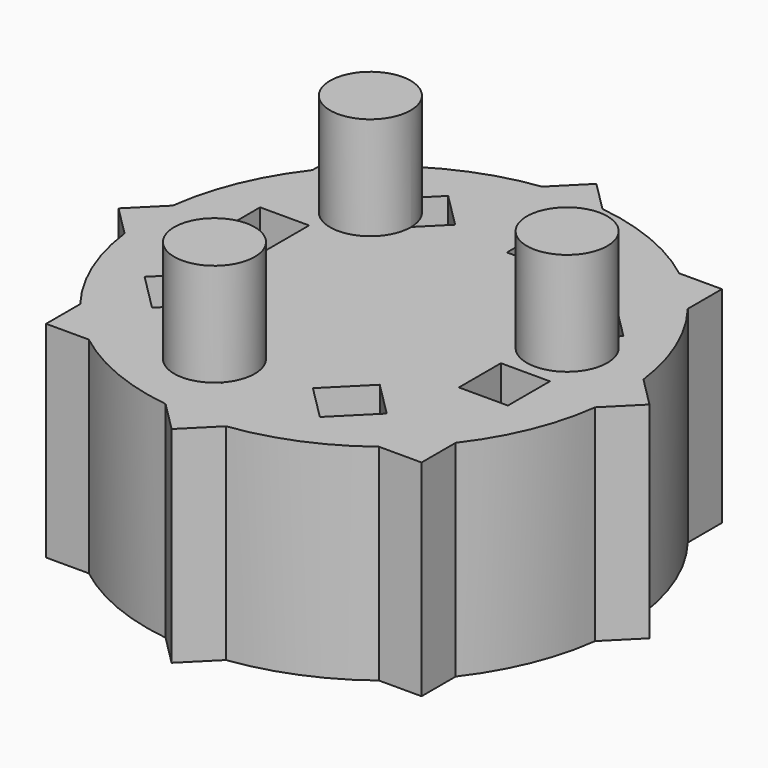
from build123d import *

# Parameters (mm, degrees)
F0_R            = 58.5548573359
F1_DEPTH        = 25.4
F2_R            = 9.9387856365
F3_DEPTH        = 25.4
F3_COPIES_COUNT = 3
F5_DEPTH        = 50.8
F5_COPIES_COUNT = 8
F6_W            = 12.9660330713
F6_H            = 12.1016278863
F7_DEPTH        = 25.4
F7_COPIES_COUNT = 8


# Not quite as in the source:
# - a pattern or mirror of a feature is missing from the dataset's text; its kind, count and spacing are read off the source's solid


with BuildPart() as f1:
    # F0 (on Top) → F1 (new body, symmetric)
    with BuildSketch(Plane.XY):
        Circle(F0_R)
    extrude(amount=F1_DEPTH, both=True)

    # F2 (on face) → F3 (join)
    with BuildSketch(Plane.XY.offset(25.4)):
        with Locations((-26.5582595021, 29.0003977716)):
            Circle(F2_R)
    f3 = extrude(amount=F3_DEPTH)

    # F3_copies: F3 ×3 about axis
    f3_copies_axis = Axis((0, 0, 0), (0, 0, 1))
    for i in range(1, F3_COPIES_COUNT):
        add(f3.rotate(f3_copies_axis, i * 360 / F3_COPIES_COUNT))

    # F4 (on face) → F5 (join, through all)
    with BuildSketch(Plane.XY.offset(25.4)):
        with BuildLine():
            Line((0, 65.528380896), (-7.4493038573, 58.0790770387))
            ThreePointArc((-7.4493038573, 58.0790770387), (0, 58.5548573359), (7.4493038573, 58.0790770387))
            Line((7.4493038573, 58.0790770387), (0, 65.528380896))
        make_face()
    f5 = extrude(amount=-F5_DEPTH)

    # F5_copies: F5 ×8 about axis
    f5_copies_axis = Axis((0, 0, 0), (0, 0, 1))
    for i in range(1, F5_COPIES_COUNT):
        add(f5.rotate(f5_copies_axis, i * 360 / F5_COPIES_COUNT))

    # F6 (on face) → F7 (cut)
    with BuildSketch(Plane.XY.offset(25.4)):
        with Locations((10.9036043286, 38.4410806)):
            Rectangle(F6_W, F6_H)
    f7 = extrude(amount=-F7_DEPTH, mode=Mode.SUBTRACT)

    # F7_copies: F7 ×8 about axis
    f7_copies_axis = Axis((0, 0, 0), (0, 0, 1))
    for i in range(1, F7_COPIES_COUNT):
        add(f7.rotate(f7_copies_axis, i * 360 / F7_COPIES_COUNT), mode=Mode.SUBTRACT)


solid = f1.part
